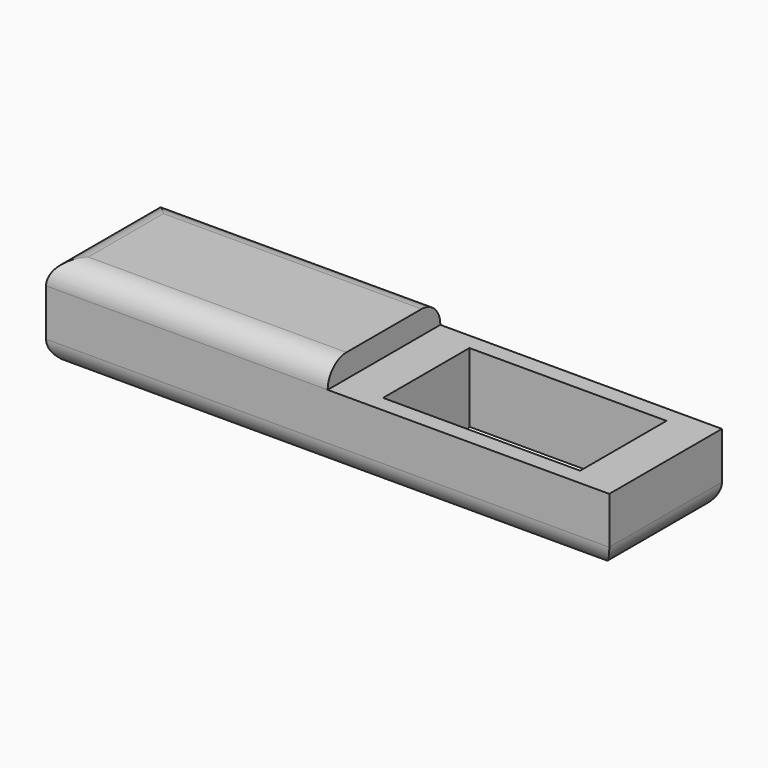
from build123d import *

# Parameters (mm, degrees)
F0_W        = 120
F0_H        = 30
F1_DEPTH    = 20
F3_DEPTH    = 25
F4_DEPTH    = 5
F5_T1_DEPTH = 85
F5_T3_DEPTH = 145
F5_T5_DEPTH = 55


# Not quite as in the source:
# - a fillet or chamfer that OpenCascade refuses, or shapes differently, is made with other operations: its cross-section is extruded or revolved along the edge and cut away or added


with BuildPart() as f1:
    # F0 (on Top) → F1 (new body)
    with BuildSketch(Plane.XY):
        Rectangle(F0_W, F0_H)
    extrude(amount=F1_DEPTH)

    # F2 (on face) → F3 (cut)
    with BuildSketch(Plane.XY.offset(20)):
        Polygon((9, 11.5), (9, 0), (30, 0), (51, 0), (51, 11.5), align=None)
        Polygon((30, 0), (9, 0), (9, -11.5), (51, -11.5), (51, 0), align=None)
    extrude(amount=-F3_DEPTH, mode=Mode.SUBTRACT)

    # F2 (on face) → F4 (cut)
    with BuildSketch(Plane.XY.offset(20)):
        Polygon((0, 15), (0, 0), (9, 0), (9, 11.5), (51, 11.5), (51, 0), (60, 0), (60, 15), align=None)
        Polygon((9, 0), (0, 0), (0, -15), (60, -15), (60, 0), (51, 0), (51, -11.5), (9, -11.5), align=None)
    extrude(amount=-F4_DEPTH, mode=Mode.SUBTRACT)

    # F5: fillet of radius 5 on 7 edges, made by hand

    # F5_s2 → F5_t1 (cut)
    with BuildSketch(Plane.YZ.offset(-72.5)):
        with BuildLine():
            ThreePointArc((-15, 15), (-13.5355339059, 18.5355339059), (-10, 20))
            Line((-10, 20), (-15, 20))
            Line((-15, 20), (-15, 15))
        make_face()
        with BuildLine():
            ThreePointArc((15, 15), (13.5355339059, 18.5355339059), (10, 20))
            Line((10, 20), (15, 20))
            Line((15, 20), (15, 15))
        make_face()
    extrude(amount=F5_T1_DEPTH, mode=Mode.SUBTRACT)

    # F5_s4 → F5_t3 (cut)
    with BuildSketch(Plane.YZ.offset(-72.5)):
        with BuildLine():
            ThreePointArc((-10, 0), (-13.5355339059, 1.4644660941), (-15, 5))
            Line((-15, 5), (-15, 0))
            Line((-15, 0), (-10, 0))
        make_face()
        with BuildLine():
            ThreePointArc((10, 0), (13.5355339059, 1.4644660941), (15, 5))
            Line((15, 5), (15, 0))
            Line((15, 0), (10, 0))
        make_face()
    extrude(amount=F5_T3_DEPTH, mode=Mode.SUBTRACT)

    # F5_s6 → F5_t5 (cut)
    with BuildSketch(Plane.XZ.offset(-27.5)):
        with BuildLine():
            ThreePointArc((60, 5), (58.5355339059, 1.4644660941), (55, 0))
            Line((55, 0), (60, 0))
            Line((60, 0), (60, 5))
        make_face()
        with BuildLine():
            ThreePointArc((-55, 0), (-58.5355339059, 1.4644660941), (-60, 5))
            Line((-60, 5), (-60, 0))
            Line((-60, 0), (-55, 0))
        make_face()
        with BuildLine():
            ThreePointArc((-60, 15), (-58.5355339059, 18.5355339059), (-55, 20))
            Line((-55, 20), (-60, 20))
            Line((-60, 20), (-60, 15))
        make_face()
    extrude(amount=F5_T5_DEPTH, mode=Mode.SUBTRACT)


solid = f1.part
